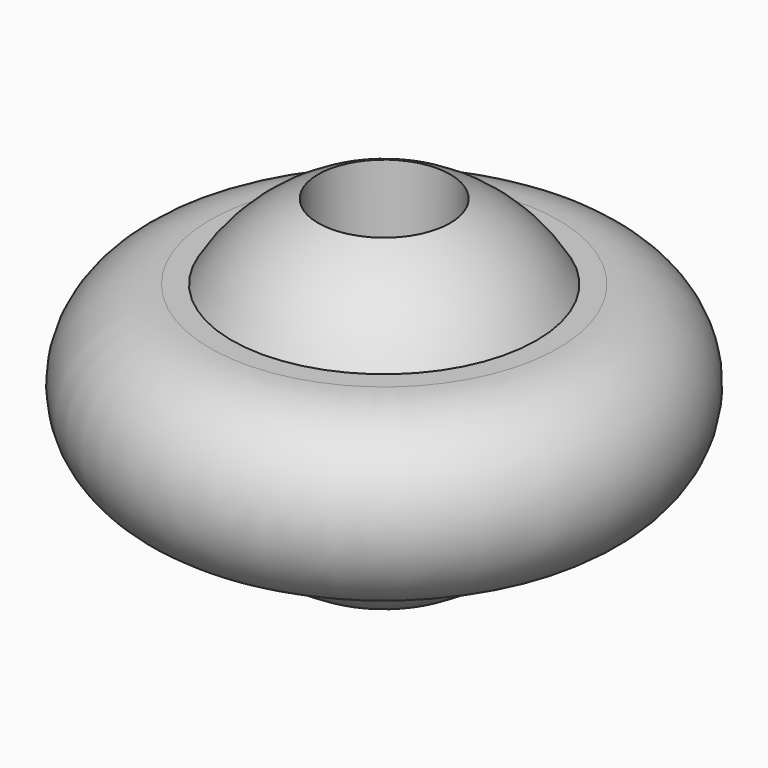
from build123d import *

# Parameters (mm, degrees)
F2_R          = 1.5
F3_DEPTH      = 3.998497265
F3_DEPTH_BACK = 4.0006311494


with BuildPart() as f1:
    # F0 (on Front) → F1 (revolve)
    with BuildSketch(Plane.XZ):
        with BuildLine():
            Line((-3.878140574, -1.9962841181), (-3.4647271293, -1.9964134512))
            ThreePointArc((-3.4647271293, -1.9964134512), (-2.0005418335, -3.4612859959), (0, -3.997497265))
            Line((0, -3.997497265), (0, 3.9996311494))
            ThreePointArc((0, 3.9996311494), (-2.000079858, 3.4636866573), (-3.4641938241, 1.9994714302))
            Line((-3.4641938241, 1.9994714302), (-3.9530518044, 1.9994488908))
            ThreePointArc((-3.9530518044, 1.9994488908), (-5.9981910715, 0.0850437646), (-4.1231084445, -1.9962074819))
            Line((-4.1231084445, -1.9962074819), (-3.878140574, -1.9962841181))
        make_face()
        with BuildLine():
            ThreePointArc((-4.1231084445, -1.9962074819), (-4.0006256837, -1.9999999021), (-3.878140574, -1.9962841181))
            Line((-3.878140574, -1.9962841181), (-4.1231084445, -1.9962074819))
        make_face()
    revolve(axis=Axis((0, 0, 0.0010669422), (0, 0, -1)))

    # F2 (on Top) → F3 (cut, two sides)
    with BuildSketch(Plane.XY) as f3_sk:
        Circle(F2_R)
    extrude(amount=-F3_DEPTH, mode=Mode.SUBTRACT)
    extrude(f3_sk.sketch, amount=F3_DEPTH_BACK, mode=Mode.SUBTRACT)


solid = f1.part
